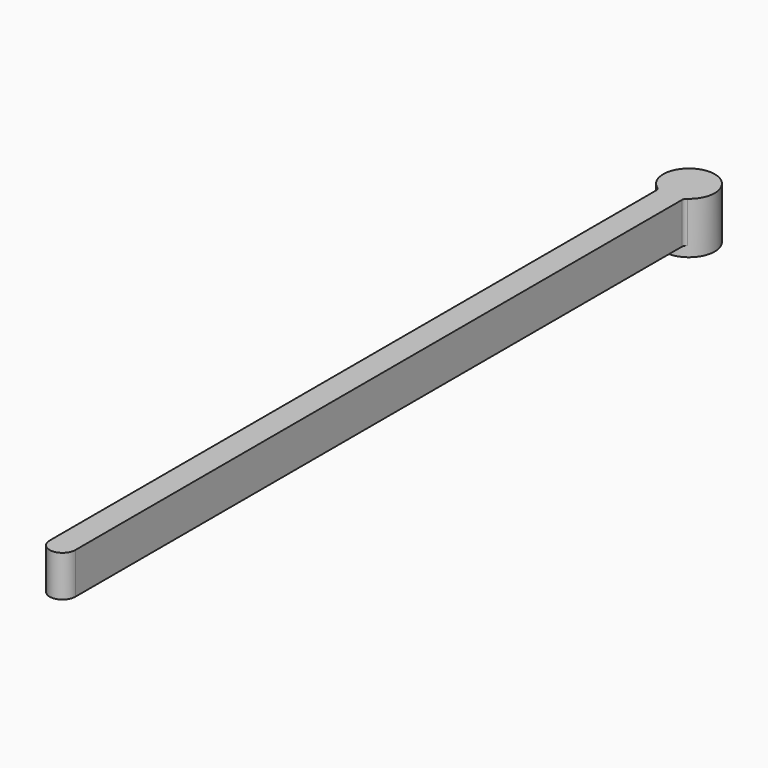
from build123d import *
from build123d import SkipClean  # not in build123d's __all__

# Parameters (mm, degrees)
F1_DEPTH = 8
F2_DEPTH = 2
F3_R     = 1


with BuildPart() as f1:
    # F0 (on Top) → F1 (new body)
    with BuildSketch(Plane.XY):
        with BuildLine():
            ThreePointArc((17.5, -23.4724675501), (20, -24.1423405312), (22.5, -23.4724675501))
            ThreePointArc((22.5, -23.4724675501), (24.3301270189, -21.6423405312), (25, -19.1423405312))
            ThreePointArc((25, -19.1423405312), (17.5, -14.8122135123), (17.5, -23.4724675501))
        make_face()
        with BuildLine():
            ThreePointArc((17.5, -46.837484988), (20.0298455202, -45.8127197232), (22.5, -44.6514277487))
            Line((22.5, -44.6514277487), (22.5, -40.3887360535))
            Line((22.5, -40.3887360535), (22.5, -23.4724675501))
            ThreePointArc((22.5, -23.4724675501), (20, -24.1423405312), (17.5, -23.4724675501))
            Line((17.5, -23.4724675501), (17.5, -46.837484988))
        make_face()
        with BuildLine():
            Line((22.5, -171.3366569068), (22.5, -44.6514277487))
            ThreePointArc((22.5, -44.6514277487), (20.0298455202, -45.8127197232), (17.5, -46.837484988))
            Line((17.5, -46.837484988), (17.5, -171.3366569068))
            Line((17.5, -171.3366569068), (22.5, -171.3366569068))
        make_face()
        with BuildLine():
            ThreePointArc((17.5, -171.3366569068), (20, -173.8366569068), (22.5, -171.3366569068))
            Line((22.5, -171.3366569068), (17.5, -171.3366569068))
        make_face()
    extrude(amount=F1_DEPTH)

    # F0 (on Top) → F2 (join)
    with BuildSketch(Plane.XY):
        with BuildLine():
            ThreePointArc((17.5, -23.4724675501), (20, -24.1423405312), (22.5, -23.4724675501))
            ThreePointArc((22.5, -23.4724675501), (24.3301270189, -21.6423405312), (25, -19.1423405312))
            ThreePointArc((25, -19.1423405312), (17.5, -14.8122135123), (17.5, -23.4724675501))
        make_face()
    with SkipClean():  # cleaning this boolean's faces spoils the solid; the shape is the same uncleaned
        extrude(amount=-F2_DEPTH)

    # F3#2 (call 1 of 2: OpenCascade refuses the feature's edges together)
    f3_2_edges = [f1.edges().sort_by_distance(p)[0] for p in [
        (22.5, -23.472468, 4),
    ]]
    fillet(f3_2_edges, radius=F3_R)

    # F3 (call 2 of 2)
    f3_edges = [f1.edges().sort_by_distance(p)[0] for p in [
        (17.5, -23.472468, 4),
    ]]
    fillet(f3_edges, radius=F3_R)


solid = f1.part
